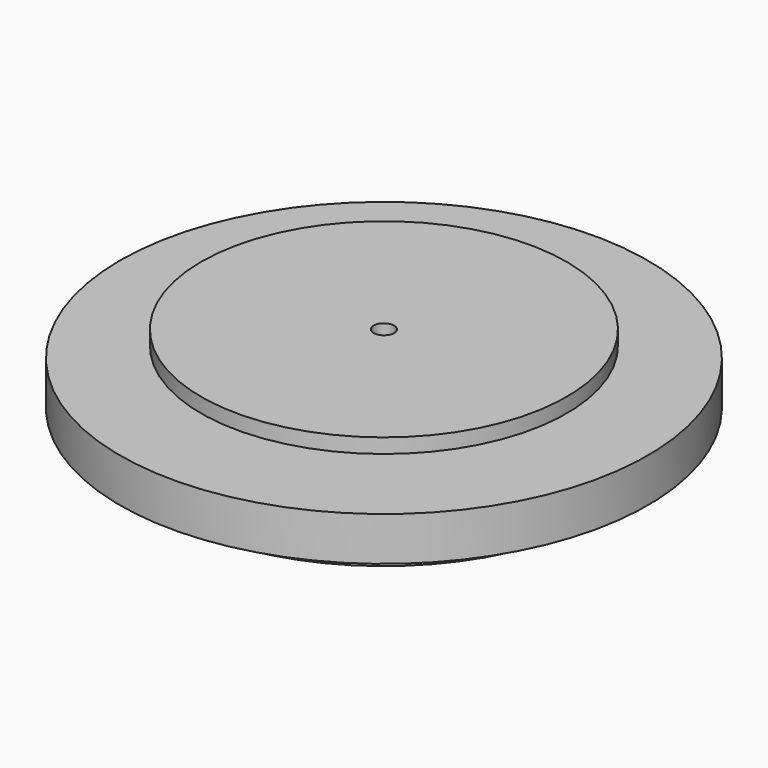
from build123d import *

# Parameters (mm, degrees)
F0_W            = 25
F0_H            = 6
F2_W            = 1.1
F2_H            = 7.7406916718
F3_DEPTH        = 110
F3_COPIES_COUNT = 3


# Not quite as in the source:
# - an extrude ends at something that could not be found from the text; its depth is read off the source's solid
# - a pattern or mirror of a feature is missing from the dataset's text; its kind, count and spacing are read off the source's solid


with BuildPart() as f1:
    # F0 (on Front) → F1 (revolve)
    with BuildSketch(Plane.XZ):
        Polygon((-1.4, -12.9), (-1.4, 0), (-25, 0), (-25, -2), (-5.8, -2), (-5.8, -2.8), (-2.7, -2.8), (-2.7, -12.2242640687), (-3.2, -12.7242640687), (-3.2, -13.0014611872), (-1.4, -14.0406916718), align=None)
    revolve(axis=Axis((0, 0, -0.0521782535), (0, 0, -1)))

    # F2 (on Right) → F3 (cut, through all)
    with BuildSketch(Plane.YZ):
        with Locations((0, -10.1703458359)):
            Rectangle(F2_W, F2_H)
    f3 = extrude(amount=F3_DEPTH, mode=Mode.SUBTRACT)

    # F3_copies: F3 ×3 about axis
    f3_copies_axis = Axis((0, 0, 0), (0, 0, 1))
    for i in range(1, F3_COPIES_COUNT):
        add(f3.rotate(f3_copies_axis, i * 360 / F3_COPIES_COUNT), mode=Mode.SUBTRACT)


with BuildPart() as f1b:
    # F0 (on Front) → F1, piece 2 (revolve)
    with BuildSketch(Plane.XZ):
        Polygon((-3.8, -12.9), (-3, -12.1), (-3, -3), (-3.8, -3), (-3.8, -10.1), (-5.8, -10.1), (-5.8, -10.9), (-30, -10.9), (-30, -12.9), align=None)
    revolve(axis=Axis((0, 0, -0.0521782535), (0, 0, -1)))


with BuildPart() as f1c:
    # F0 (on Front) → F1, piece 3 (revolve)
    with BuildSketch(Plane.XZ):
        with Locations((-23.6, -6.45)):
            Rectangle(F0_W, F0_H)
    revolve(axis=Axis((0, 0, -0.0521782535), (0, 0, -1)))


solid = Compound([f1.part, f1b.part, f1c.part])
